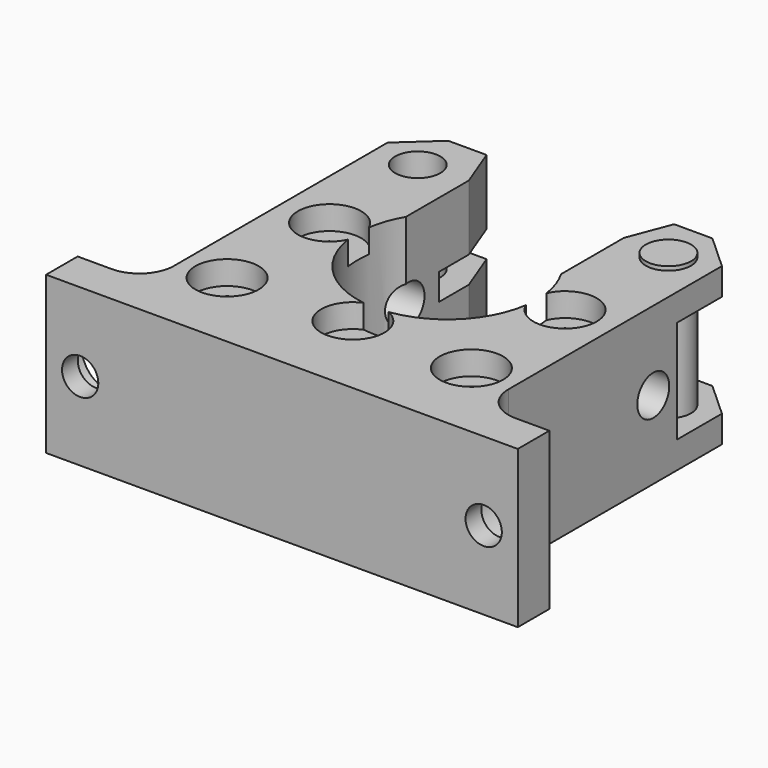
from build123d import *
from build123d import SkipClean  # not in build123d's __all__

# Parameters (mm, degrees)
F1_DEPTH       = 19.88
F2_R           = 4.382
F3_R           = 3.81
F4_DEPTH       = 2.5
F4_DEPTH_BACK  = 5
F5_R           = 2.2987
F6_DEPTH       = 2.501
F7_R           = 4.01
F8_DEPTH       = 3
F9_R           = 1.8288
F10_DEPTH      = 19.8810001
F11_R          = 2.53
F12_DEPTH      = 21.176
F14_W          = 12.0765847373
F14_H          = 13.03
F15_DEPTH      = 11.351
F16_W          = 10.5
F16_H          = 3.36
F17_DEPTH      = 11.351
F18_R          = 2.865
F19_DEPTH      = 20
F19_DEPTH_BACK = 0.5
F20_R          = 2.865
F21_DEPTH      = 20.001


# Not quite as in the source:
# - after a boolean that leaves OpenCascade's solid faulty, fix() repairs it


with BuildPart() as f1:
    # F0 (on Top) → F1 (new body)
    with BuildSketch(Plane.XY):
        with BuildLine():
            Line((0, -11.375), (0, -26.185))
            Line((0, -26.185), (29.875, -26.185))
            Line((29.875, -26.185), (29.875, -21.185))
            Line((29.875, -21.185), (21.175, -21.185))
            Line((21.175, -21.185), (21.175, 17.015))
            Line((21.175, 17.015), (16.7292900036, 21.065))
            Line((16.7292900036, 21.065), (11.8792900036, 21.065))
            Line((11.8792900036, 21.065), (9.825, 15.6823642592))
            Line((9.825, 15.6823642592), (9.825, 5.7323642592))
            ThreePointArc((9.825, 5.7323642592), (9.8639816618, -5.6650234577), (0, -11.375))
        make_face()
    extrude(amount=F1_DEPTH)

    # F2
    f2_edges = [f1.edges().sort_by_distance(p)[0] for p in [
        (21.175, -21.185, 9.94),
    ]]
    fillet(f2_edges, radius=F2_R)

    # F3 (on face) → F4 (cut, two sides)
    with BuildSketch(Plane(origin=(0, -21.185, 0), x_dir=(-1, 0, 0), z_dir=(0, 1, 0))) as f4_sk:
        with Locations((-25.557, 9.94)):
            Circle(F3_R)
    extrude(amount=-F4_DEPTH, mode=Mode.SUBTRACT)
    extrude(f4_sk.sketch, amount=F4_DEPTH_BACK, mode=Mode.SUBTRACT)

    # F5 (on face) → F6 (cut, through all)
    with BuildSketch(Plane(origin=(0, -23.685, 0), x_dir=(-1, 0, 0), z_dir=(0, 1, 0))):
        with Locations((-25.557, 9.94)):
            Circle(F5_R)
    extrude(amount=-F6_DEPTH, mode=Mode.SUBTRACT)

    # F7 (on face) → F8 (cut)
    with BuildSketch(Plane.XY.offset(19.88)):
        with Locations((15.475, -15.525)):
            Circle(F7_R)
        with Locations((0, -14.955)):
            Circle(F7_R)
        with Locations((14.915, 0)):
            Circle(F7_R)
    extrude(amount=-F8_DEPTH, mode=Mode.SUBTRACT)

    # F9 (on face) → F10 (cut, through all)
    with BuildSketch(Plane.XY.offset(19.88)):
        with Locations((14.915, 0)):
            Circle(F9_R)
        with Locations((15.475, -15.525)):
            Circle(F9_R)
        with Locations((0, -14.955)):
            Circle(F9_R)
    extrude(amount=-F10_DEPTH, mode=Mode.SUBTRACT)

    # F11 (on face) → F12 (cut, through all)
    with BuildSketch(Plane.YZ.offset(21.175)):
        with Locations((6.145, 9.89)):
            Circle(F11_R)
    extrude(amount=-F12_DEPTH, mode=Mode.SUBTRACT)

    # F13: F1 across plane


with BuildPart() as f1_1:
    add(f1.part, clean=False)
    with SkipClean():  # cleaning this boolean's faces spoils the solid; the shape is the same uncleaned
        add(f1.part.mirror(Plane.YZ), clean=False)

    # F14 (on face) → F15 (cut, through all)
    with BuildSketch(Plane.YZ.offset(21.175)):
        with Locations((15.9632923686, 9.94)):
            Rectangle(F14_W, F14_H)
    extrude(amount=-F15_DEPTH, mode=Mode.SUBTRACT)

    add(f1_1.part.fix(), mode=Mode.REPLACE)

    # F16 (on face) → F17 (cut, through all)
    with BuildSketch(Plane(origin=(-21.175, 0, 0), x_dir=(0, -1, 0), z_dir=(-1, 0, 0))):
        with Locations((-16.215, 9.94)):
            Rectangle(F16_W, F16_H)
    extrude(amount=-F17_DEPTH, mode=Mode.SUBTRACT)

    # F18 (on face) → F19 (join, two sides)
    with BuildSketch(Plane.XY.offset(19.88)) as f19_sk:
        with Locations((15.875, 15.17)):
            Circle(F18_R)
    extrude(amount=-F19_DEPTH)
    extrude(f19_sk.sketch, amount=F19_DEPTH_BACK)

    # F20 (on face) → F21 (cut, through all)
    with BuildSketch(Plane.XY.offset(19.88)):
        with Locations((-15.875, 15.17)):
            Circle(F20_R)
    extrude(amount=-F21_DEPTH, mode=Mode.SUBTRACT)


solid = f1_1.part
